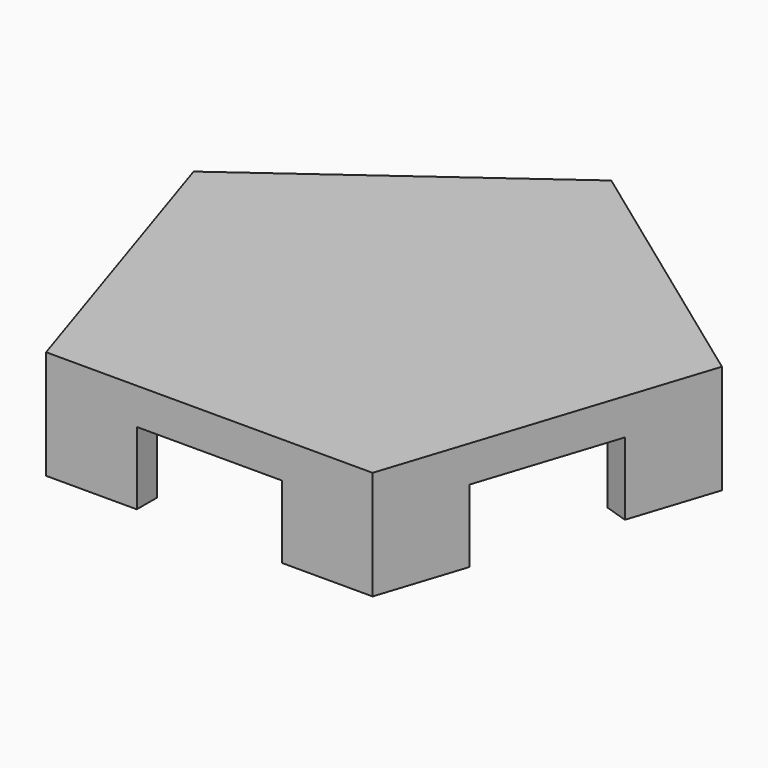
from build123d import *

# Parameters (mm, degrees)
F1_DEPTH = 7.62
F3_DEPTH = 5.08
F4_W     = 10.16
F4_H     = 1.748005039
F5_DEPTH = 5.08


# Not quite as in the source:
# - a feature names something its author has since deleted; it is built from what else it names


with BuildPart() as f1:
    # F0 (on Top) → F1 (new body)
    with BuildSketch(Plane.XY):
        Polygon((-11.43, -15.732045351), (11.43, -15.732045351), (18.4941284914, 6.0091066115), (0, 19.4458774789), (-18.4941284914, 6.0091066115), align=None)
    extrude(amount=F1_DEPTH)

    # F2 (on Top) → F3 (cut)
    with BuildSketch(Plane.XY):
        Polygon((10.16, -13.984040312), (16.4392253257, 5.3414280991), (0, 17.2852244257), (-16.4392253257, 5.3414280991), (-10.16, -13.984040312), align=None)
    extrude(amount=F3_DEPTH, mode=Mode.SUBTRACT)

    # F4 (on face) → F5 (cut)
    with BuildSketch(Plane(origin=(0, 0, 0), x_dir=(1, 0, 0), z_dir=(0, 0, -1))):
        Polygon((-14.8694189943, -0.5100609964), (-13.2996126628, 4.3213061064), (-14.9620642457, 4.8614693697), (-16.5318705771, 0.030102267), align=None)
        Polygon((-14.9620642457, 4.8614693697), (-13.2996126628, 4.3213061064), (-11.7298063314, 9.1526732092), (-13.3922579143, 9.6928364725), align=None)
        Polygon((11.7298063314, 9.1526732092), (13.2996126628, 4.3213061064), (14.9620642457, 4.8614693697), (13.3922579143, 9.6928364725), align=None)
        Polygon((14.9620642457, 4.8614693697), (13.2996126628, 4.3213061064), (14.8694189943, -0.5100609964), (16.5318705771, 0.030102267), align=None)
        with Locations((0, 14.8580428315)):
            Rectangle(F4_W, F4_H)
        Polygon((0, -19.4458774789), (0, -17.2852244257), (-11.3019674114, -9.0738644512), (-12.3294189943, -10.488030234), align=None)
        Polygon((11.3019674114, -9.0738644512), (0, -17.2852244257), (0, -19.4458774789), (12.3294189943, -10.488030234), align=None)
    extrude(amount=-F5_DEPTH, mode=Mode.SUBTRACT)


solid = f1.part
